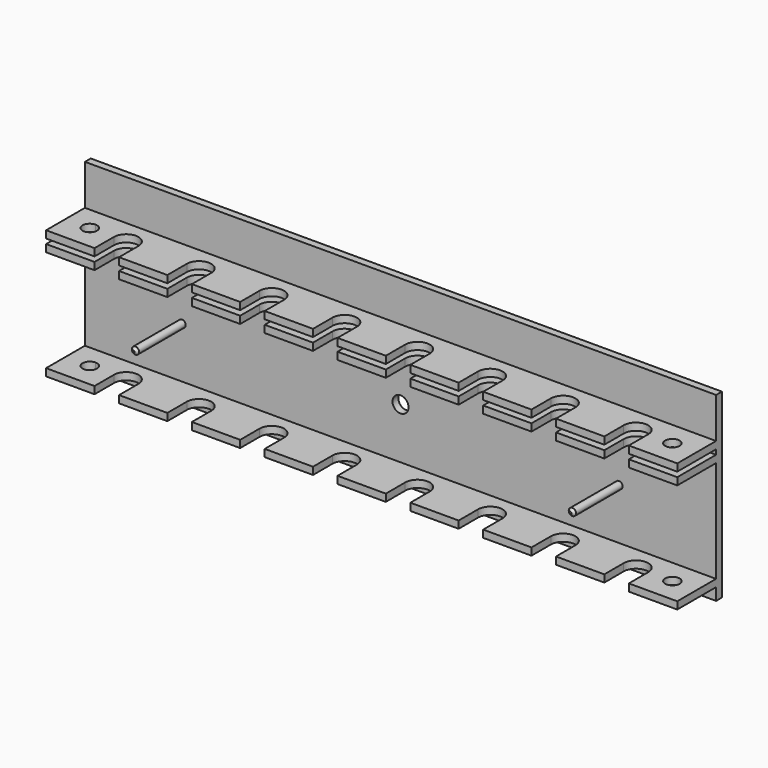
from build123d import *

# Parameters (mm, degrees)
F0_W      = 30
F0_H      = 20
F1_DEPTH  = 3
F2_W      = 30
F2_H      = 21.6892715544
F2_H_2    = 3
F2_H_3    = 50
F3_DEPTH  = 3
F4_W      = 30
F4_H      = 3
F5_DEPTH  = 20
F10_W     = 240
F10_H     = 23
F11_DEPTH = 3
F12_W     = 10.1
F12_H     = 10
F13_DEPTH = 72
F15_D     = 6.6
F15_DEPTH = 21.5
F15_TIP   = 1.9828400428
F16_R     = 1.5
F17_DEPTH = 25
F18_SIZE  = 1
F20_DEPTH = 10
F22_DEPTH = 10
F23_R     = 3
F24_DEPTH = 60


# Not quite as in the source:
# - a feature names something its author has since deleted; it is built from what else it names


with BuildPart() as f1:
    # F0 (on Top) → F1 (new body)
    with BuildSketch(Plane.XY):
        Rectangle(F0_W, F0_H)
    extrude(amount=-F1_DEPTH)

    # F2 (on face) → F3 (join)
    with BuildSketch(Plane(origin=(0, 10, 0), x_dir=(-1, 0, 0), z_dir=(0, 1, 0))):
        with Locations((0, 10.8446357772)):
            Rectangle(F2_W, F2_H)
        with Locations((0, -1.5)):
            Rectangle(F2_W, F2_H_2)
        with Locations((0, -28)):
            Rectangle(F2_W, F2_H_3)
    extrude(amount=F3_DEPTH)

    # F4 (on face) → F5 (join)
    with BuildSketch(Plane.XZ.offset(-10)):
        with Locations((0, 3.5)):
            Rectangle(F4_W, F4_H)
    extrude(amount=F5_DEPTH)

    # F6: F1 across face


with BuildPart() as f1_1:
    add(f1.part)
    add(f1.part.mirror(Plane(origin=(15, 7.489162772, -9.8464985819), x_dir=(0, 1, 0), z_dir=(1, 0, 0))))

    # F7: F1 across face


with BuildPart() as f1_2:
    add(f1_1.part)
    add(f1_1.part.mirror(Plane(origin=(45, 7.489162772, -9.8464985819), x_dir=(0, 1, 0), z_dir=(1, 0, 0))))

    # F8: F1 across face


with BuildPart() as f1_3:
    add(f1_2.part)
    add(f1_2.part.mirror(Plane(origin=(105, 7.489162772, -9.8464985819), x_dir=(0, 1, 0), z_dir=(1, 0, 0))))

    # F10 (on offset) → F11 (join)
    with BuildSketch(Plane(origin=(0, 0, -48), x_dir=(1, 0, 0), z_dir=(0, 0, -1))):
        with Locations((105, -1.5)):
            Rectangle(F10_W, F10_H)
    extrude(amount=-F11_DEPTH)

    # F12 (on face) → F13 (cut)
    with BuildSketch(Plane(origin=(0, 0, -48), x_dir=(1, 0, 0), z_dir=(0, 0, -1))):
        with Locations((0, 5)):
            Rectangle(F12_W, F12_H)
        with BuildLine():
            Line((5.05, 0), (-5.05, 0))
            ThreePointArc((-5.05, 0), (0, -5.05), (5.05, 0))
        make_face()
        with BuildLine():
            Line((35.05, 10), (24.95, 10))
            Line((24.95, 10), (24.95, 0))
            ThreePointArc((24.95, 0), (30, -5.05), (35.05, 0))
            Line((35.05, 0), (35.05, 10))
        make_face()
        with BuildLine():
            Line((65.05, 10), (54.95, 10))
            Line((54.95, 10), (54.95, 0))
            ThreePointArc((54.95, 0), (60, -5.05), (65.05, 0))
            Line((65.05, 0), (65.05, 10))
        make_face()
        with BuildLine():
            Line((95.05, 10), (84.95, 10))
            Line((84.95, 10), (84.95, 0))
            ThreePointArc((84.95, 0), (90, -5.05), (95.05, 0))
            Line((95.05, 0), (95.05, 10))
        make_face()
        with BuildLine():
            Line((125.05, 10), (114.95, 10))
            Line((114.95, 10), (114.95, 0))
            ThreePointArc((114.95, 0), (120, -5.05), (125.05, 0))
            Line((125.05, 0), (125.05, 10))
        make_face()
        with BuildLine():
            Line((155.05, 0), (155.05, 10))
            Line((155.05, 10), (144.95, 10))
            Line((144.95, 10), (144.95, 0))
            ThreePointArc((144.95, 0), (150, -5.05), (155.05, 0))
        make_face()
        with BuildLine():
            Line((185.05, 0), (185.05, 10))
            Line((185.05, 10), (174.95, 10))
            Line((174.95, 10), (174.95, 0))
            ThreePointArc((174.95, 0), (180, -5.05), (185.05, 0))
        make_face()
        with BuildLine():
            Line((215.05, 0), (215.05, 10))
            Line((215.05, 10), (204.95, 10))
            Line((204.95, 10), (204.95, 0))
            ThreePointArc((204.95, 0), (210, -5.05), (215.05, 0))
        make_face()
    extrude(amount=-F13_DEPTH, mode=Mode.SUBTRACT)

    # F15
    with Locations(Plane.XZ.offset(-10)):
        with Locations((105, -24)):
            Hole(F15_D / 2, depth=F15_DEPTH)
            with Locations((0, 0, -(F15_DEPTH + F15_TIP / 2))):  # 118° drill point
                Cone(0, F15_D / 2, F15_TIP, mode=Mode.SUBTRACT)

    # F16 (on face) → F17 (join)
    with BuildSketch(Plane.XZ.offset(-10)):
        with Locations((15, -24)):
            Circle(F16_R)
        with Locations((195, -24)):
            Circle(F16_R)
    extrude(amount=F17_DEPTH)

    # F18
    f18_edges = [f1_3.edges().sort_by_distance(p)[0] for p in [
        (13.5, -15, -24),
        (193.5, -15, -24),
    ]]
    chamfer(f18_edges, length=F18_SIZE)

    # F19 (on face) → F20 (join)
    with BuildSketch(Plane.YZ.offset(225)):
        Polygon((13, 21.6892715544), (10, 21.6892715544), (10, 5), (-10, 5), (-10, 2), (10, 2), (10, 0), (-10, 0), (-10, -3), (10, -3), (10, -45), (-10, -45), (-10, -48), (10, -48), (10, -53), (13, -53), align=None)
    extrude(amount=F20_DEPTH)

    # F21 (on face) → F22 (join)
    with BuildSketch(Plane(origin=(-15, 0, 0), x_dir=(0, -1, 0), z_dir=(-1, 0, 0))):
        Polygon((-10, 5), (-10, 21.6892715544), (-13, 21.6892715544), (-13, -53), (-10, -53), (-10, -48), (10, -48), (10, -45), (-10, -45), (-10, -3), (10, -3), (10, 0), (-10, 0), (-10, 2), (10, 2), (10, 5), align=None)
    extrude(amount=F22_DEPTH)

    # F23 (on face) → F24 (cut)
    with BuildSketch(Plane.XY.offset(5)):
        with BuildLine():
            ThreePointArc((-15, -3), (-12.8786796564, -2.1213203436), (-12, 0))
            ThreePointArc((-12, 0), (-12.8786796564, 2.1213203436), (-15, 3))
            Line((-15, 3), (-15, -3))
        make_face()
        with BuildLine():
            Line((-15, -3), (-15, 3))
            ThreePointArc((-15, 3), (-18, 0), (-15, -3))
        make_face()
        with Locations((225, 0)):
            Circle(F23_R)
    extrude(amount=-F24_DEPTH, mode=Mode.SUBTRACT)


solid = f1_3.part
